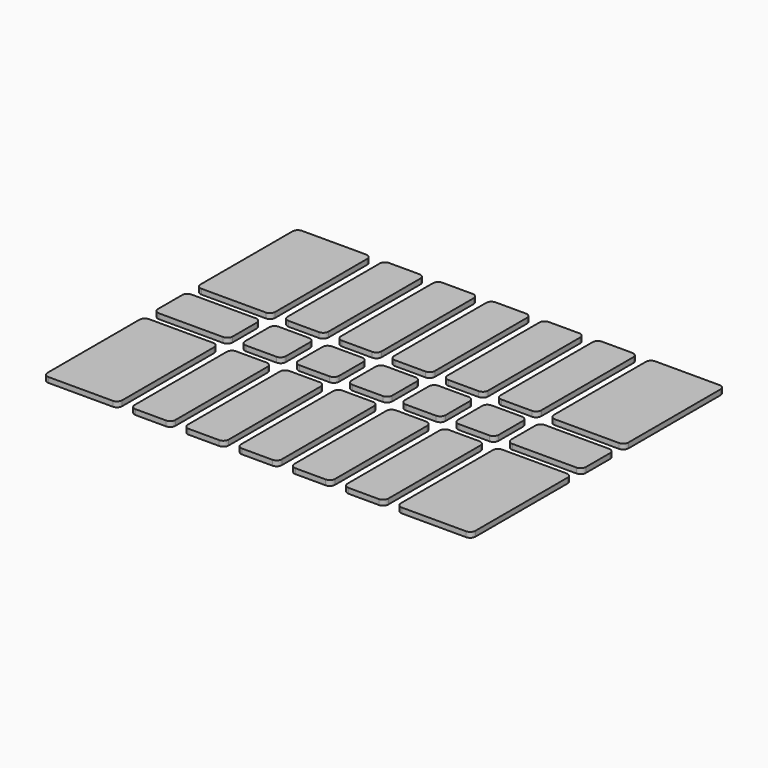
from build123d import *

# Parameters (mm, degrees)
F1_DEPTH = 1


with BuildPart() as f1:
    # F0 (on Top) → F1 (new body)
    with BuildSketch(Plane.XY):
        with BuildLine():
            Line((-27.7, -6.3), (-40, -6.3))
            ThreePointArc((-40, -6.3), (-40.7071067812, -6.5928932188), (-41, -7.3))
            Line((-41, -7.3), (-41, -29.35))
            ThreePointArc((-41, -29.35), (-40.7071067812, -30.0571067812), (-40, -30.35))
            Line((-40, -30.35), (-27.7, -30.35))
            ThreePointArc((-27.7, -30.35), (-26.9928932188, -30.0571067812), (-26.7, -29.35))
            Line((-26.7, -29.35), (-26.7, -7.3))
            ThreePointArc((-26.7, -7.3), (-26.9928932188, -6.5928932188), (-27.7, -6.3))
        make_face()
    extrude(amount=F1_DEPTH)


with BuildPart() as f1b:
    # F0 (on Top) → F1, piece 2 (new body)
    with BuildSketch(Plane.XY):
        with BuildLine():
            Line((-17.5, -6.3), (-23.3, -6.3))
            ThreePointArc((-23.3, -6.3), (-24.0071067812, -6.5928932188), (-24.3, -7.3))
            Line((-24.3, -7.3), (-24.3, -29.35))
            ThreePointArc((-24.3, -29.35), (-24.0071067812, -30.0571067812), (-23.3, -30.35))
            Line((-23.3, -30.35), (-17.5, -30.35))
            ThreePointArc((-17.5, -30.35), (-16.7928932188, -30.0571067812), (-16.5, -29.35))
            Line((-16.5, -29.35), (-16.5, -7.3))
            ThreePointArc((-16.5, -7.3), (-16.7928932188, -6.5928932188), (-17.5, -6.3))
        make_face()
    extrude(amount=F1_DEPTH)


with BuildPart() as f1c:
    # F0 (on Top) → F1, piece 3 (new body)
    with BuildSketch(Plane.XY):
        with BuildLine():
            Line((-7.3, -6.3), (-13.1, -6.3))
            ThreePointArc((-13.1, -6.3), (-13.8071067812, -6.5928932188), (-14.1, -7.3))
            Line((-14.1, -7.3), (-14.1, -29.35))
            ThreePointArc((-14.1, -29.35), (-13.8071067812, -30.0571067812), (-13.1, -30.35))
            Line((-13.1, -30.35), (-7.3, -30.35))
            ThreePointArc((-7.3, -30.35), (-6.5928932188, -30.0571067812), (-6.3, -29.35))
            Line((-6.3, -29.35), (-6.3, -7.3))
            ThreePointArc((-6.3, -7.3), (-6.5928932188, -6.5928932188), (-7.3, -6.3))
        make_face()
    extrude(amount=F1_DEPTH)


with BuildPart() as f1d:
    # F0 (on Top) → F1, piece 4 (new body)
    with BuildSketch(Plane.XY):
        with BuildLine():
            Line((2.9, -6.3), (-2.9, -6.3))
            ThreePointArc((-2.9, -6.3), (-3.6071067812, -6.5928932188), (-3.9, -7.3))
            Line((-3.9, -7.3), (-3.9, -29.35))
            ThreePointArc((-3.9, -29.35), (-3.6071067812, -30.0571067812), (-2.9, -30.35))
            Line((-2.9, -30.35), (2.9, -30.35))
            ThreePointArc((2.9, -30.35), (3.6071067812, -30.0571067812), (3.9, -29.35))
            Line((3.9, -29.35), (3.9, -7.3))
            ThreePointArc((3.9, -7.3), (3.6071067812, -6.5928932188), (2.9, -6.3))
        make_face()
    extrude(amount=F1_DEPTH)


with BuildPart() as f1e:
    # F0 (on Top) → F1, piece 5 (new body)
    with BuildSketch(Plane.XY):
        with BuildLine():
            Line((-27.7, 3.9), (-40, 3.9))
            ThreePointArc((-40, 3.9), (-40.7071067812, 3.6071067812), (-41, 2.9))
            Line((-41, 2.9), (-41, -2.9))
            ThreePointArc((-41, -2.9), (-40.7071067812, -3.6071067812), (-40, -3.9))
            Line((-40, -3.9), (-27.7, -3.9))
            ThreePointArc((-27.7, -3.9), (-26.9928932188, -3.6071067812), (-26.7, -2.9))
            Line((-26.7, -2.9), (-26.7, 2.9))
            ThreePointArc((-26.7, 2.9), (-26.9928932188, 3.6071067812), (-27.7, 3.9))
        make_face()
    extrude(amount=F1_DEPTH)


with BuildPart() as f1f:
    # F0 (on Top) → F1, piece 6 (new body)
    with BuildSketch(Plane.XY):
        with BuildLine():
            Line((-17.5, 3.9), (-23.3, 3.9))
            ThreePointArc((-23.3, 3.9), (-24.0071067812, 3.6071067812), (-24.3, 2.9))
            Line((-24.3, 2.9), (-24.3, -2.9))
            ThreePointArc((-24.3, -2.9), (-24.0071067812, -3.6071067812), (-23.3, -3.9))
            Line((-23.3, -3.9), (-17.5, -3.9))
            ThreePointArc((-17.5, -3.9), (-16.7928932188, -3.6071067812), (-16.5, -2.9))
            Line((-16.5, -2.9), (-16.5, 2.9))
            ThreePointArc((-16.5, 2.9), (-16.7928932188, 3.6071067812), (-17.5, 3.9))
        make_face()
    extrude(amount=F1_DEPTH)


with BuildPart() as f1g:
    # F0 (on Top) → F1, piece 7 (new body)
    with BuildSketch(Plane.XY):
        with BuildLine():
            Line((-7.3, 3.9), (-13.1, 3.9))
            ThreePointArc((-13.1, 3.9), (-13.8071067812, 3.6071067812), (-14.1, 2.9))
            Line((-14.1, 2.9), (-14.1, -2.9))
            ThreePointArc((-14.1, -2.9), (-13.8071067812, -3.6071067812), (-13.1, -3.9))
            Line((-13.1, -3.9), (-7.3, -3.9))
            ThreePointArc((-7.3, -3.9), (-6.5928932188, -3.6071067812), (-6.3, -2.9))
            Line((-6.3, -2.9), (-6.3, 2.9))
            ThreePointArc((-6.3, 2.9), (-6.5928932188, 3.6071067812), (-7.3, 3.9))
        make_face()
    extrude(amount=F1_DEPTH)


with BuildPart() as f1h:
    # F0 (on Top) → F1, piece 8 (new body)
    with BuildSketch(Plane.XY):
        with BuildLine():
            Line((2.9, 3.9), (-2.9, 3.9))
            ThreePointArc((-2.9, 3.9), (-3.6071067812, 3.6071067812), (-3.9, 2.9))
            Line((-3.9, 2.9), (-3.9, -2.9))
            ThreePointArc((-3.9, -2.9), (-3.6071067812, -3.6071067812), (-2.9, -3.9))
            Line((-2.9, -3.9), (2.9, -3.9))
            ThreePointArc((2.9, -3.9), (3.6071067812, -3.6071067812), (3.9, -2.9))
            Line((3.9, -2.9), (3.9, 2.9))
            ThreePointArc((3.9, 2.9), (3.6071067812, 3.6071067812), (2.9, 3.9))
        make_face()
    extrude(amount=F1_DEPTH)


with BuildPart() as f2_1:
    # F2: instance of F1
    add(f1.part.mirror(Plane.XZ))


with BuildPart() as f2_2:
    # F2: instance of F1b
    add(f1b.part.mirror(Plane.XZ))


with BuildPart() as f2_3:
    # F2: instance of F1c
    add(f1c.part.mirror(Plane.XZ))


with BuildPart() as f2_4:
    # F2: instance of F1d
    add(f1d.part.mirror(Plane.XZ))


with BuildPart() as f3_1:
    # F3: instance of F2_1
    add(f2_1.part.mirror(Plane.YZ))


with BuildPart() as f3_2:
    # F3: instance of F2_2
    add(f2_2.part.mirror(Plane.YZ))


with BuildPart() as f3_3:
    # F3: instance of F2_3
    add(f2_3.part.mirror(Plane.YZ))


with BuildPart() as f3_4:
    # F3: instance of F1g
    add(f1g.part.mirror(Plane.YZ))


with BuildPart() as f3_5:
    # F3: instance of F1f
    add(f1f.part.mirror(Plane.YZ))


with BuildPart() as f3_6:
    # F3: instance of F1e
    add(f1e.part.mirror(Plane.YZ))


with BuildPart() as f3_7:
    # F3: instance of F1
    add(f1.part.mirror(Plane.YZ))


with BuildPart() as f3_8:
    # F3: instance of F1b
    add(f1b.part.mirror(Plane.YZ))


with BuildPart() as f3_9:
    # F3: instance of F1c
    add(f1c.part.mirror(Plane.YZ))


solid = Compound([f1.part, f1b.part, f1c.part, f1d.part, f1e.part, f1f.part, f1g.part, f1h.part, f2_1.part, f2_2.part, f2_3.part, f2_4.part, f3_1.part, f3_2.part, f3_3.part, f3_4.part, f3_5.part, f3_6.part, f3_7.part, f3_8.part, f3_9.part])
